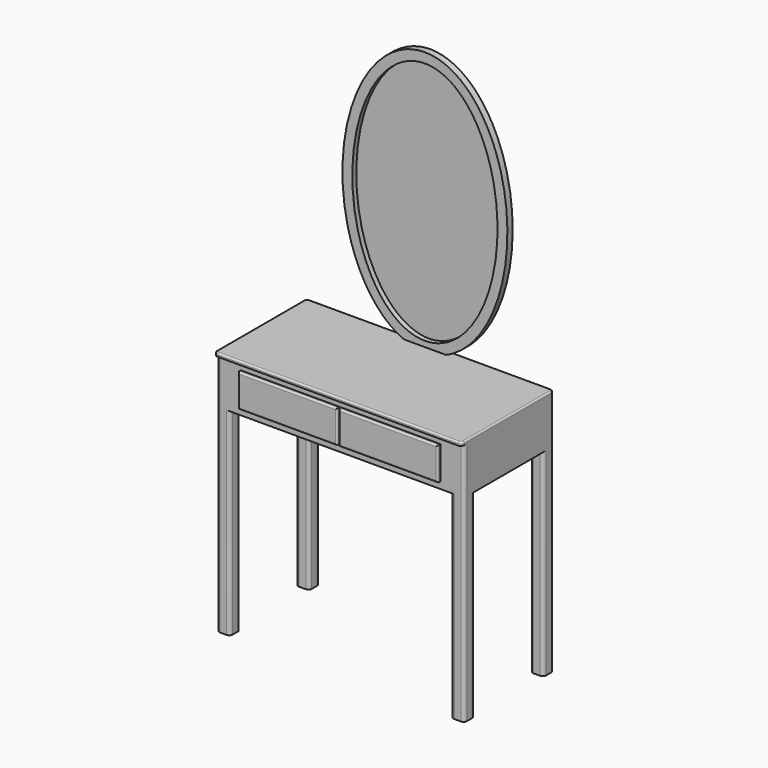
from build123d import *

# Parameters (mm, degrees)
F1_DEPTH  = 350
F2_W      = 260
F2_H      = 610
F3_DEPTH  = 750.001
F4_W      = 300
F4_H      = 100
F5_DEPTH  = 10
F6_R      = 9.9999
F7_R      = 5
F8_R      = 5
F10_DEPTH = 5
F11_DEPTH = 20


# Not quite as in the source:
# - a fillet or chamfer is up to 0.001 mm smaller than in the source, because OpenCascade refuses the exact size


with BuildPart() as f1:
    # F0 (on Front) → F1 (new body)
    with BuildSketch(Plane.XZ):
        Polygon((375, 750), (-375, 750), (-375, 600), (-375, 0), (-335, 0), (-335, 600), (335, 600), (335, 0), (375, 0), (375, 600), align=None)
    extrude(amount=F1_DEPTH)

    # F2 (on face) → F3 (cut, through all)
    with BuildSketch(Plane.YZ.offset(375)):
        with Locations((-170, 295)):
            Rectangle(F2_W, F2_H)
    extrude(amount=-F3_DEPTH, mode=Mode.SUBTRACT)

    # F4 (on face) → F5 (cut)
    with BuildSketch(Plane.XZ.offset(350)):
        Polygon((375, 740), (-375, 740), (-375, 0), (-335, 0), (-335, 600), (335, 600), (335, 0), (375, 0), align=None)
        with Locations((-152.5, 670)):
            Rectangle(F4_W, F4_H, mode=Mode.SUBTRACT)
        with Locations((152.5, 670)):
            Rectangle(F4_W, F4_H, mode=Mode.SUBTRACT)
    extrude(amount=-F5_DEPTH, mode=Mode.SUBTRACT)

    # F6 (radius 10 in the source; OpenCascade refuses exactly that, so slightly less here)
    f6_edges = [f1.edges().sort_by_distance(p)[0] for p in [
        (-375, 0, 375),
        (-375, -340, 370),
        (375, -340, 370),
        (375, 0, 375),
        (335, -40, 300),
        (335, 0, 300),
        (375, -40, 300),
        (-335, 0, 300),
        (-335, -40, 300),
        (-375, -40, 300),
        (375, -300, 300),
        (335, -300, 300),
        (335, -340, 300),
        (-335, -340, 300),
        (-335, -300, 300),
        (-375, -300, 300),
        (375, -350, 745),
        (-375, -350, 745),
    ]]
    fillet(f6_edges, radius=F6_R)

    # F7
    f7_edges = [f1.edges().sort_by_distance(p)[0] for p in [
        (152.5, -350, 620),
        (302.5, -350, 670),
        (152.5, -350, 720),
        (2.5, -350, 670),
        (-2.5, -350, 670),
        (-152.5, -350, 620),
        (-302.5, -350, 670),
        (-152.5, -350, 720),
    ]]
    fillet(f7_edges, radius=F7_R)

    # F8
    f8_edges = [f1.edges().sort_by_distance(p)[0] for p in [
        (0, -350, 750),
    ]]
    fillet(f8_edges, radius=F8_R)



with BuildPart() as f10:
    # F9 (on face) → F10 (new body)
    with BuildSketch(Plane(origin=(0, 0, 0), x_dir=(-1, 0, 0), z_dir=(0, 1, 0))):
        with BuildLine():
            add(Edge.make_bspline(
                [(0, 766.9183588453), (381.0511776652, 766.9183588453), (190.5255888326, 1321.9183588453), (0, 1876.9183588453), (-190.5255888326, 1321.9183588453), (-381.0511776652, 766.9183588453), (0, 766.9183588453)],
                knots=[0, 0, 0, 2.0943951024, 2.0943951024, 4.1887902048, 4.1887902048, 6.2831853072, 6.2831853072, 6.2831853072], degree=2, weights=[1, 0.5, 1, 0.5, 1, 0.5, 1]))
        make_face()
    extrude(amount=-F10_DEPTH)


with BuildPart() as f1_1:
    add(f1.part)

    add(f10.part)  # F11 merges F10
    # F9 (on face) → F11 (join)
    with BuildSketch(Plane(origin=(0, 0, 0), x_dir=(-1, 0, 0), z_dir=(0, 1, 0))):
        with BuildLine():
            Line((-50, 745), (50, 745))
            add(Edge.make_bspline(
                [(50, 745), (415.2704758851, 864.2968378696), (207.6352379426, 1359.7013842068), (0, 1855.1059305439), (-207.6352379426, 1359.7013842068), (-415.2704758851, 864.2968378696), (-50, 745)],
                knots=[0.2013579208, 0.2013579208, 0.2013579208, 2.1615144093, 2.1615144093, 4.1216708979, 4.1216708979, 6.0818273864, 6.0818273864, 6.0818273864], degree=2, weights=[1, 0.5569575634, 1, 0.5569575634, 1, 0.5569575634, 1]))
        make_face()
        with BuildLine():
            add(Edge.make_bspline(
                [(0, 766.9183588453), (381.0511776652, 766.9183588453), (190.5255888326, 1321.9183588453), (0, 1876.9183588453), (-190.5255888326, 1321.9183588453), (-381.0511776652, 766.9183588453), (0, 766.9183588453)],
                knots=[0, 0, 0, 2.0943951024, 2.0943951024, 4.1887902048, 4.1887902048, 6.2831853072, 6.2831853072, 6.2831853072], degree=2, weights=[1, 0.5, 1, 0.5, 1, 0.5, 1]))
        make_face(mode=Mode.SUBTRACT)
    extrude(amount=-F11_DEPTH)


solid = f1_1.part
